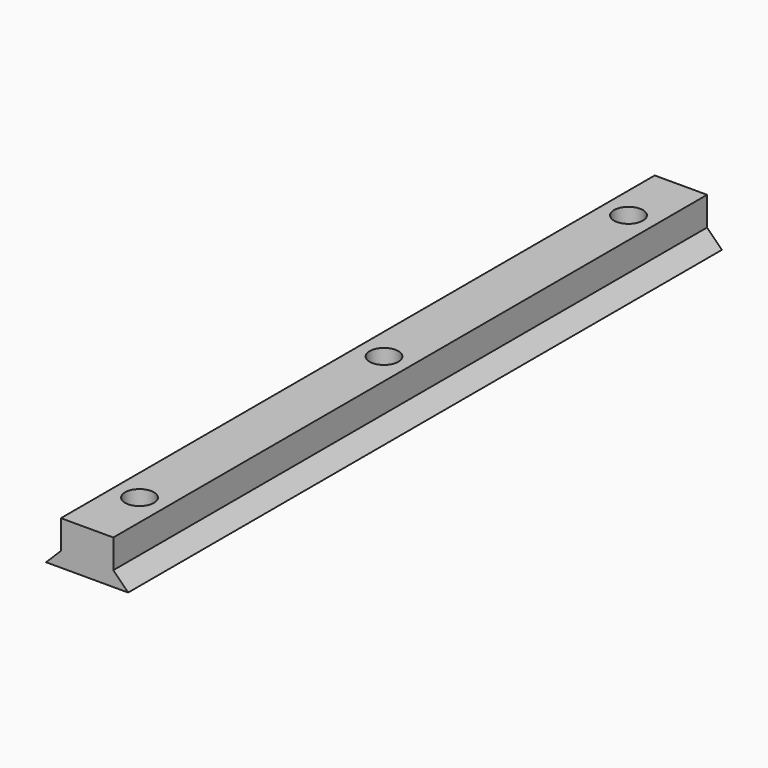
from build123d import *

# Parameters (mm, degrees)
F0_W           = 6
F0_H           = 3.3
F1_DEPTH       = 42.5
F3_D           = 3.3
F3_CSINK_D     = 6.72
F3_CSINK_ANGLE = 90


with BuildPart() as f1:
    # F0 (on Front) → F1 (new body, symmetric)
    with BuildSketch(Plane.XZ):
        Rectangle(F0_W, F0_H)
        Polygon((4.7, -3.35), (3, -1.65), (-3, -1.65), (-4.7, -3.35), align=None)
    extrude(amount=F1_DEPTH, both=True)

    # F3 (through all)
    with Locations(Plane(origin=(0, 0, -3.35), x_dir=(1, 0, 0), z_dir=(0, 0, -1))):
        with Locations((0, 0), (0, 35), (0, -35)):
            CounterSinkHole(F3_D / 2, F3_CSINK_D / 2, counter_sink_angle=F3_CSINK_ANGLE)


solid = f1.part
